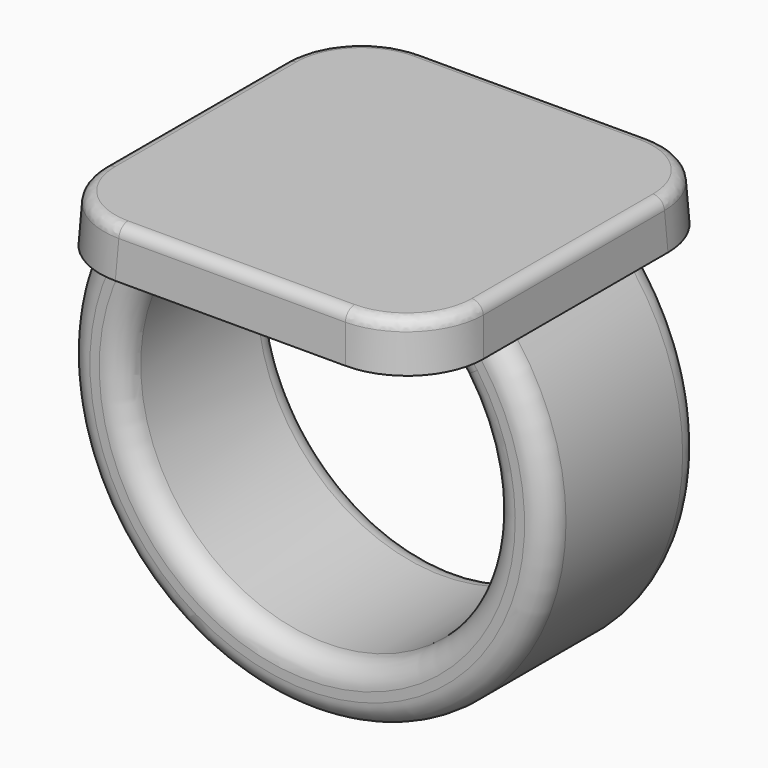
from build123d import *

# Parameters (mm, degrees)
F0_W          = 25.4
F0_H          = 25.4
F1_DEPTH      = 3.175
F1_TAPER      = 3
F3_W          = 5.08
F3_H          = 12.7
F6_DEPTH      = 6.35
F6_DEPTH_BACK = 6.35
F7_R          = 5.08
F8_R          = 1.524
F9_R          = 0.762


with BuildPart() as f1:
    # F0 (on Top) → F1 (new body)
    with BuildSketch(Plane.XY):
        Rectangle(F0_W, F0_H)
    extrude(amount=F1_DEPTH, taper=F1_TAPER)

    # F4: sweep along a path in F2
    with BuildLine(Plane.XZ) as f4_path:
        ThreePointArc((-10.16, 0), (0, -23.5582897328), (10.16, 0))
    # F3 (on face) → F4 (sweep)
    with BuildSketch(Plane(origin=(0, 0, 0), x_dir=(1, 0, 0), z_dir=(0, 0, -1))):
        with Locations((-10.16, 0)):
            Rectangle(F3_W, F3_H)
    sweep(path=f4_path.line)

    # F5 (on Front) → F6 (join, two sides)
    with BuildSketch(Plane.XZ) as f6_sk:
        with BuildLine():
            ThreePointArc((7.62, 0), (8.9072265211, -1.1822790439), (10.0130578512, -2.535746045))
            Line((10.0130578512, -2.535746045), (10.16, 0))
            Line((10.16, 0), (7.62, 0))
        make_face()
    extrude(amount=F6_DEPTH)
    extrude(f6_sk.sketch, amount=-F6_DEPTH_BACK)

    # F7
    f7_edges = [f1.edges().sort_by_distance(p)[0] for p in [
        (12.616803, -12.616803, 1.5875),
        (-12.616803, -12.616803, 1.5875),
        (-12.616803, 12.616803, 1.5875),
        (12.616803, 12.616803, 1.5875),
    ]]
    fillet(f7_edges, radius=F7_R)

    # F8
    f8_edges = [f1.edges().sort_by_distance(p)[0] for p in [
        (-1.743325, 6.35, -21.711017),
        (-1.743325, -6.35, -21.711017),
        (8.907227, -6.35, -1.182279),
        (0, -6.35, -25.501344),
        (0, 6.35, -25.501344),
        (8.907227, 6.35, -1.182279),
    ]]
    fillet(f8_edges, radius=F8_R)

    # F9
    f9_edges = [f1.edges().sort_by_distance(p)[0] for p in [
        (12.533605, 0, 3.175),
        (11.048589, -11.048589, 3.175),
        (11.048589, 11.048589, 3.175),
        (0, -12.533605, 3.175),
        (0, 12.533605, 3.175),
        (-11.048589, -11.048589, 3.175),
        (-11.048589, 11.048589, 3.175),
        (-12.533605, 0, 3.175),
    ]]
    fillet(f9_edges, radius=F9_R)


solid = f1.part
